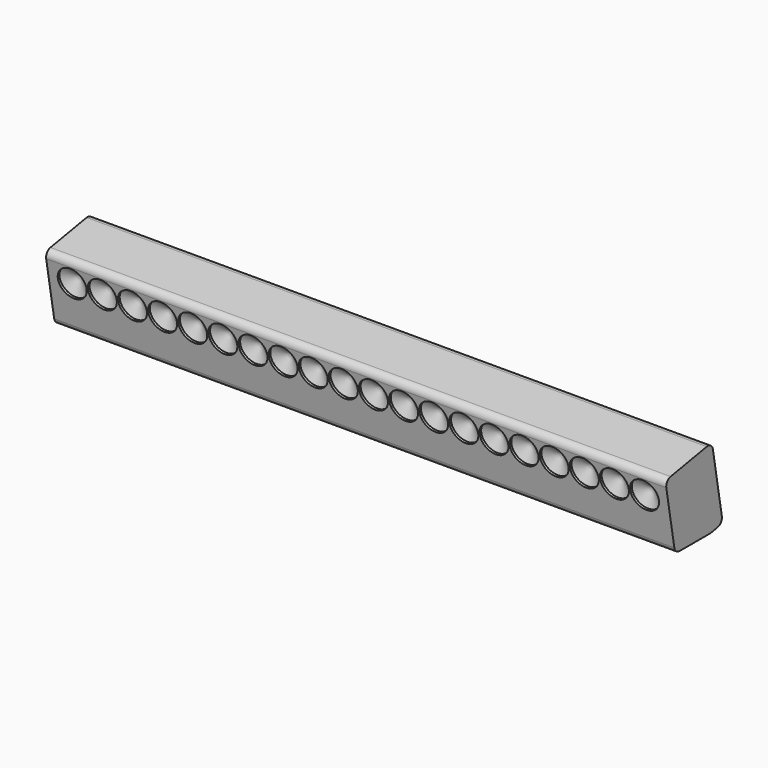
from build123d import *

# Parameters (mm, degrees)
F1_DEPTH = 700
F2_R     = 15
F4_D     = 65
F4_DEPTH = 5
F4_TIP   = 19.5279701184


# Not quite as in the source:
# - a feature names something its author has since deleted; it is built from what else it names


with BuildPart() as f1:
    # F0 (on Right) → F1 (new body, symmetric)
    with BuildSketch(Plane.YZ):
        Polygon((-27.4648018735, 155.7606315443), (0, 0), (100, 0), (134.4682713554, 6.0776862183), (103.9881005213, 178.9393249289), align=None)
    extrude(amount=F1_DEPTH, both=True)

    # F2
    f2_edges = [f1.edges().sort_by_distance(p)[0] for p in [
        (0, 100, 0),
        (0, 134.468271, 6.077686),
        (0, 103.988101, 178.939325),
        (0, -27.464802, 155.760632),
        (0, 0, 0),
    ]]
    fillet(f2_edges, radius=F2_R)

    # F4
    with Locations(Plane(origin=(0, 0, 0), x_dir=(1, 0, 0), z_dir=(0, -0.984807753, -0.1736481777))):
        with Locations((-646, 108.1634903542), (-578, 108.1634903542), (-510, 108.1634903542), (-442, 108.1634903542), (-374, 108.1634903542), (-306, 108.1634903542), (-238, 108.1634903542), (-170, 108.1634903542), (-102, 108.1634903542), (-34, 108.1634903542), (34, 108.1634903542), (102, 108.1634903542), (170, 108.1634903542), (238, 108.1634903542), (306, 108.1634903542), (374, 108.1634903542), (442, 108.1634903542), (510, 108.1634903542), (578, 108.1634903542), (646, 108.1634903542)):
            Hole(F4_D / 2, depth=F4_DEPTH)
            with Locations((0, 0, -(F4_DEPTH + F4_TIP / 2))):  # 118° drill point
                Cone(0, F4_D / 2, F4_TIP, mode=Mode.SUBTRACT)


solid = f1.part
